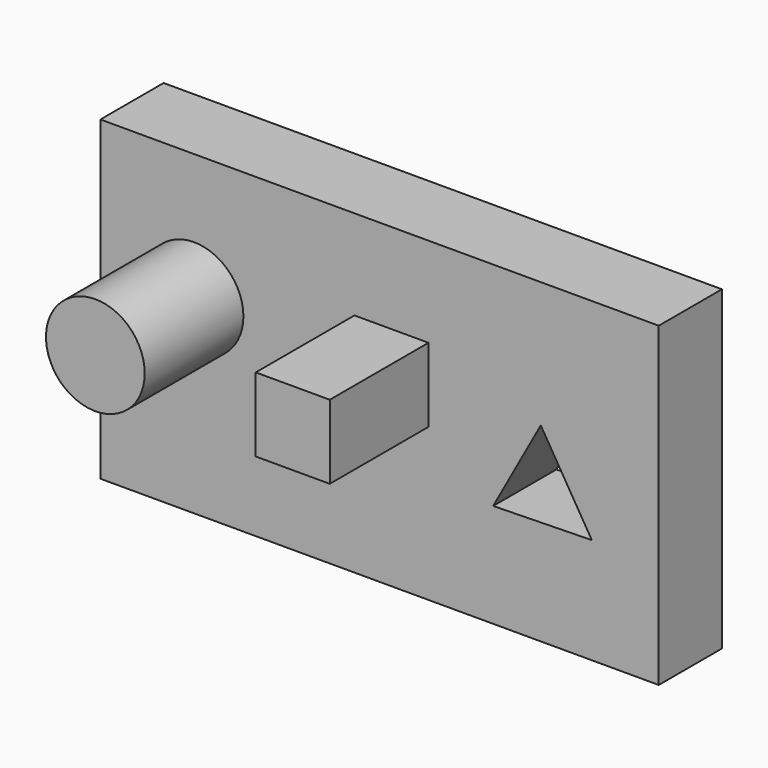
from build123d import *

# Parameters (mm, degrees)
F0_R     = 12.7
F1_DEPTH = 31.75
F0_W     = 143.6709240079
F0_H     = 81.3919715583
F2_DEPTH = 20.32


# Not quite as in the source:
# - a feature names something its author has since deleted; it is built from what else it names


with BuildPart() as f1:
    # F0 (on Front) → F1 (new body)
    with BuildSketch(Plane.XZ):
        with Locations((-82.55, 0)):
            Circle(F0_R)
    extrude(amount=F1_DEPTH)


with BuildPart() as f1b:
    # F0 (on Front) → F1, piece 2 (new body)
    with BuildSketch(Plane.XZ):
        Polygon((-31.75, 0), (-22.225, 0), (-22.225, 9.525), (-41.275, 9.525), (-41.275, 0), align=None)
        Polygon((-22.225, -9.525), (-22.225, 0), (-31.75, 0), (-41.275, 0), (-41.275, -9.525), align=None)
    extrude(amount=F1_DEPTH)


with BuildPart() as f2:
    # F0 (on Front) → F2 (new body)
    with BuildSketch(Plane.XZ):
        with Locations((-34.8065011203, -8.0374795943)):
            Rectangle(F0_W, F0_H)
        Polygon((-5.5785784244, -22.0296108979), (6.6733725689, 0.2201013892), (19.8162131398, -21.5152555605), align=None, mode=Mode.SUBTRACT)
        with Locations((-82.55, 0)):
            Circle(F0_R, mode=Mode.SUBTRACT)
        Polygon((-22.225, 9.525), (-22.225, 0), (-22.225, -9.525), (-41.275, -9.525), (-41.275, 0), (-41.275, 9.525), align=None, mode=Mode.SUBTRACT)
        with Locations((-82.55, 0)):
            Circle(F0_R)
        Polygon((-22.225, -9.525), (-22.225, 0), (-31.75, 0), (-41.275, 0), (-41.275, -9.525), align=None)
        Polygon((-31.75, 0), (-22.225, 0), (-22.225, 9.525), (-41.275, 9.525), (-41.275, 0), align=None)
    extrude(amount=-F2_DEPTH)


solid = Compound([f1.part, f1b.part, f2.part])
